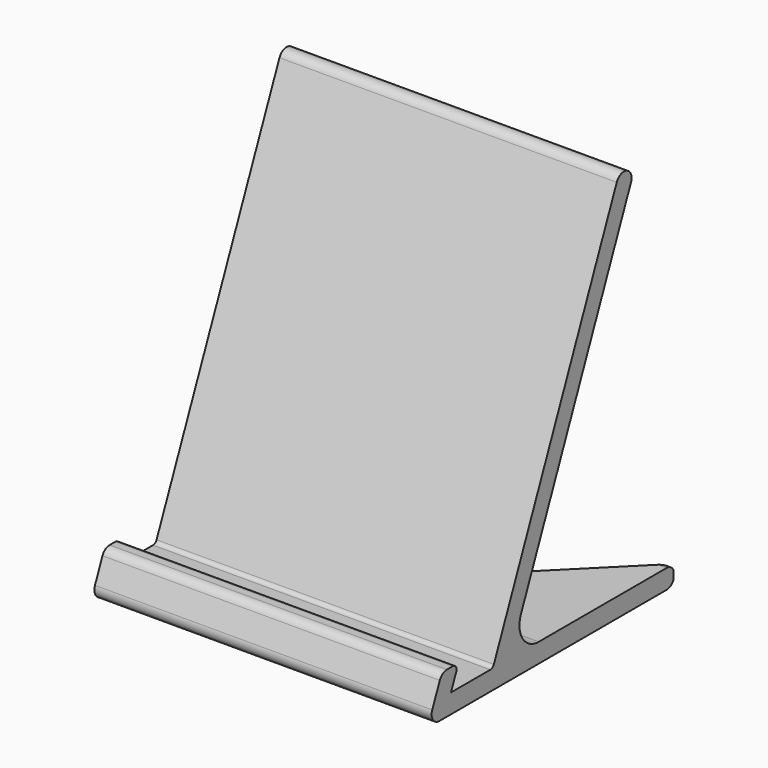
from build123d import *

# Parameters (mm, degrees)
F1_DEPTH    = 70
F2_T1_DEPTH = 80
F2_T3_DEPTH = 76.618855612
F2_T5_DEPTH = 85.1083519361
F3_R        = 1
F4_R        = 5
F6_DEPTH    = 4
F7_R        = 2
F9_DEPTH    = 1
F10_DEPTH   = 1.2
F11_R       = 1
F11_2_R     = 1


# Not quite as in the source:
# - a fillet or chamfer that OpenCascade refuses, or shapes differently, is made with other operations: its cross-section is extruded or revolved along the edge and cut away or added
# - two fillets or chamfers of one size are made in one step


with BuildPart() as f1:
    # F0 (on Right) → F1 (new body)
    with BuildSketch(Plane.YZ):
        Polygon((3.6515549073, 8.6025242673), (0, 0), (65, 0), (63.3021007352, 4), (21.2523860581, 4), (53.5124720901, 80), (49.8304526763, 81.562924514), (16.9069445485, 4), (6.0433407745, 4), (7.9969964169, 8.6025242673), align=None)
    extrude(amount=F1_DEPTH)

    # F2: fillet of radius 2 on 6 edges, made by hand

    # F2_s2 → F2_t1 (cut)
    with BuildSketch(Plane.YZ.offset(-5)):
        with BuildLine():
            ThreePointArc((51.6714623832, 80.781462257), (50.1407869393, 80.7948202592), (49.0489904193, 79.7219148071))
            Line((49.0489904193, 79.7219148071), (49.8304526763, 81.562924514))
            Line((49.8304526763, 81.562924514), (51.6714623832, 80.781462257))
        make_face()
        with BuildLine():
            ThreePointArc((52.7310098331, 78.1589902931), (52.7443678353, 79.6896657369), (51.6714623832, 80.781462257))
            Line((51.6714623832, 80.781462257), (53.5124720901, 80))
            Line((53.5124720901, 80), (52.7310098331, 78.1589902931))
        make_face()
    extrude(amount=F2_T1_DEPTH, mode=Mode.SUBTRACT)

    # F2_s4 → F2_t3 (cut)
    with BuildSketch(Plane.YZ.offset(-3.309427806)):
        with BuildLine():
            ThreePointArc((3.1343163228, 7.3839865242), (3.8714520591, 8.2702959114), (4.9753260297, 8.6025242673))
            Line((4.9753260297, 8.6025242673), (3.6515549073, 8.6025242673))
            Line((3.6515549073, 8.6025242673), (3.1343163228, 7.3839865242))
        make_face()
        with BuildLine():
            ThreePointArc((63.8193393197, 2.781462257), (63.0822035834, 3.6677716441), (61.9783296128, 4))
            Line((61.9783296128, 4), (63.3021007352, 4))
            Line((63.3021007352, 4), (63.8193393197, 2.781462257))
        make_face()
    extrude(amount=F2_T3_DEPTH, mode=Mode.SUBTRACT)

    # F2_s6 → F2_t5 (cut)
    with BuildSketch(Plane.YZ.offset(-7.5541759681)):
        with BuildLine():
            ThreePointArc((1.1806606803, 2.781462257), (1.3538987431, 0.8961260294), (3.0216703872, 0))
            Line((3.0216703872, 0), (0, 0))
            Line((0, 0), (1.1806606803, 2.781462257))
        make_face()
        with BuildLine():
            ThreePointArc((61.9783296128, 0), (63.6461012569, 0.8961260294), (63.8193393197, 2.781462257))
            Line((63.8193393197, 2.781462257), (65, 0))
            Line((65, 0), (61.9783296128, 0))
        make_face()
    extrude(amount=F2_T5_DEPTH, mode=Mode.SUBTRACT)

    # F3
    f3_edges = [f1.edges().sort_by_distance(p)[0] for p in [
        (35, 7.996996, 8.602524),
        (35, 16.906945, 4),
    ]]
    fillet(f3_edges, radius=F3_R)

    # F4
    f4_edges = [f1.edges().sort_by_distance(p)[0] for p in [
        (35, 21.252386, 4),
    ]]
    fillet(f4_edges, radius=F4_R)

    # F5 (on face) → F6 (cut, through all)
    with BuildSketch(Plane.XY.offset(4)):
        Polygon((1.8282324134, 61.9783296128), (35, 28.8065620262), (68.1717675866, 61.9783296128), (70.1717675866, 63.9783296128), (-0.1717675866, 63.9783296128), align=None)
    extrude(amount=-F6_DEPTH, mode=Mode.SUBTRACT)

    # F7
    f7_edges = [f1.edges().sort_by_distance(p)[0] for p in [
        (35, 28.806562, 2),
    ]]
    fillet(f7_edges, radius=F7_R)

    # F8 (on face) → F9 (cut)
    with BuildSketch(Plane(origin=(0, 0, 0), x_dir=(1, 0, 0), z_dir=(0, 0, -1))):
        Polygon((67.8, -5.2216703872), (2.2, -5.2216703872), (2.2, -58.495292189), (33.260303038, -27.434989151), (36.739696962, -27.434989151), (67.8, -58.495292189), align=None)
    extrude(amount=-F9_DEPTH, mode=Mode.SUBTRACT)

    # F11#2
    f11_2_edges = [f1.edges().sort_by_distance(p)[0] for p in [
        (67.8, 58.495292, 0.5),
        (67.8, 5.22167, 0.5),
        (2.2, 5.22167, 0.5),
        (2.2, 58.495292, 0.5),
        (33.260303, 27.434989, 0.5),
        (36.739697, 27.434989, 0.5),
    ]]
    fillet(f11_2_edges, radius=F11_2_R)


with BuildPart() as f10:
    # F8 (on face) → F10 (new body)
    with BuildSketch(Plane(origin=(0, 0, 0), x_dir=(1, 0, 0), z_dir=(0, 0, -1))):
        Polygon((67.8, -5.2216703872), (2.2, -5.2216703872), (2.2, -58.495292189), (33.260303038, -27.434989151), (36.739696962, -27.434989151), (67.8, -58.495292189), align=None)
    extrude(amount=F10_DEPTH)

    # F11
    f11_edges = [f10.edges().sort_by_distance(p)[0] for p in [
        (2.2, 5.22167, -0.6),
        (33.260303, 27.434989, -0.6),
        (36.739697, 27.434989, -0.6),
        (67.8, 5.22167, -0.6),
        (67.8, 58.495292, -0.6),
        (2.2, 58.495292, -0.6),
    ]]
    fillet(f11_edges, radius=F11_R)


solid = Compound([f1.part, f10.part])
